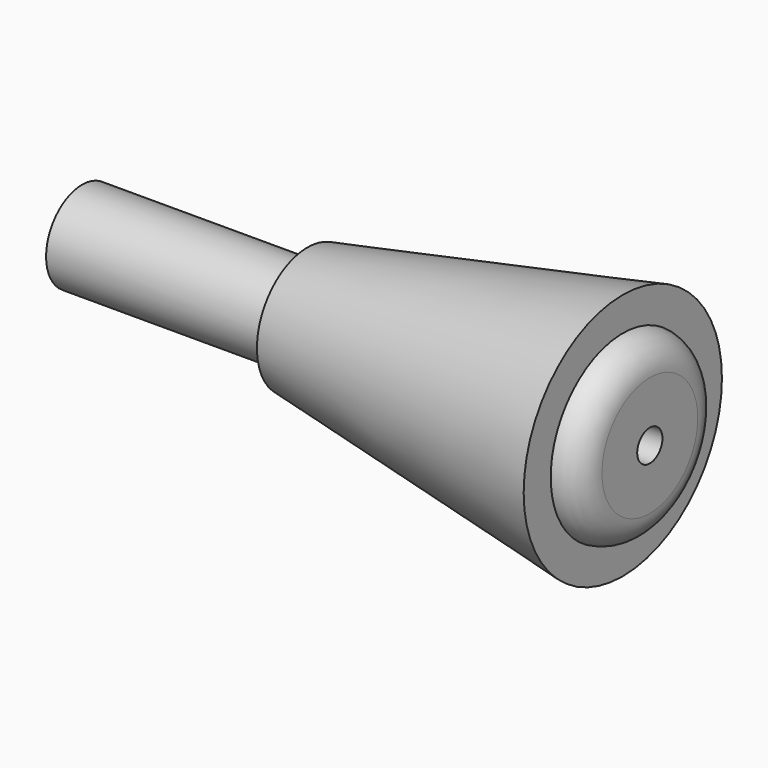
from build123d import *

# Parameters (mm, degrees)
F1_R      = 27.5
F2_R      = 14
F4_R      = 20
F5_DEPTH  = 6
F7_R      = 3.5
F8_DEPTH  = 5
F9_R      = 10
F10_DEPTH = 50
F11_DEPTH = 20


# Not quite as in the source:
# - a fillet or chamfer that OpenCascade refuses, or shapes differently, is made with other operations: its cross-section is extruded or revolved along the edge and cut away or added


with BuildPart() as f3:
    # F1 (on offset) → F3 section 0
    with BuildSketch(Plane.YZ.offset(70)):
        Circle(F1_R)
    # F2 (on Right) → F3 section 1
    with BuildSketch(Plane.YZ):
        Circle(F2_R)
    loft()

    # F4 (on face) → F5 (join)
    with BuildSketch(Plane.YZ.offset(70)):
        Circle(F4_R)
    extrude(amount=F5_DEPTH)

    # F6: fillet of radius 6.7597979746 on 1 edges, made by hand

    # F6_s1 → F6_t2 (revolve, cut)
    with BuildSketch(Plane.XY):
        with BuildLine():
            ThreePointArc((70, 20), (74.2815782992, 17.7863030167), (76, 13.2830382094))
            Line((76, 13.2830382094), (76, 20))
            Line((76, 20), (70, 20))
        make_face()
    revolve(axis=Axis((76, 0, 0), (1, 0, 0)), mode=Mode.SUBTRACT)

    # F7 (on face) → F8 (cut)
    with BuildSketch(Plane.YZ.offset(76)):
        Circle(F7_R)
    extrude(amount=-F8_DEPTH, mode=Mode.SUBTRACT)

    # F9 (on face) → F11 (cut)
    with BuildSketch(Plane(origin=(0, 0, 0), x_dir=(0, -1, 0), z_dir=(-1, 0, 0))):
        Circle(F9_R)
    extrude(amount=-F11_DEPTH, mode=Mode.SUBTRACT)


with BuildPart() as f10:
    # F9 (on face) → F10 (new body)
    with BuildSketch(Plane(origin=(0, 0, 0), x_dir=(0, -1, 0), z_dir=(-1, 0, 0))):
        Circle(F9_R)
    extrude(amount=F10_DEPTH)


solid = Compound([f3.part, f10.part])
